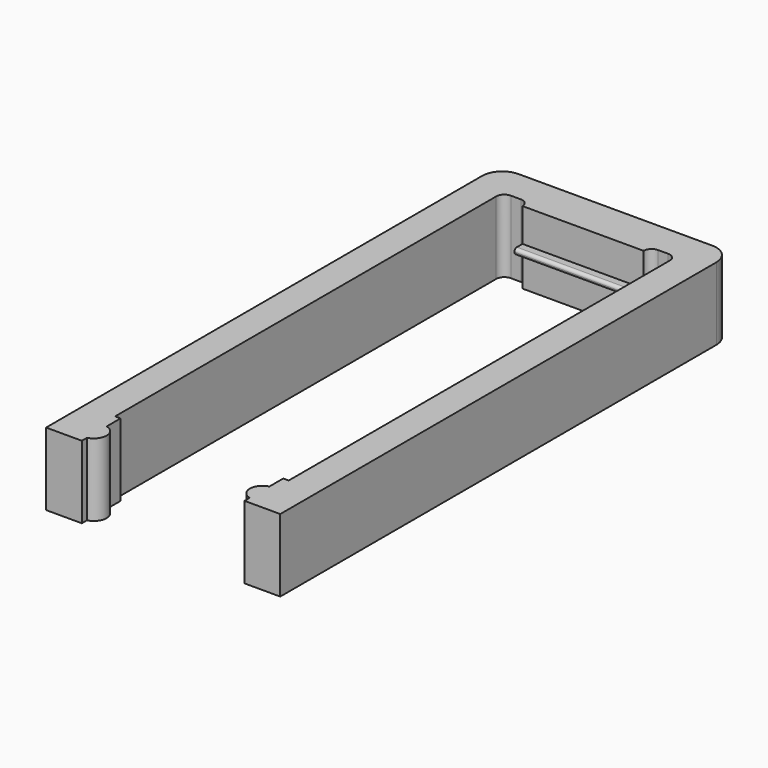
from build123d import *

# Parameters (mm, degrees)
F2_DEPTH = 18
F3_W     = 30
F3_H     = 1.5
F4_DEPTH = 2.5
F5_R     = 0.75
F6_R     = 0.74999


# Not quite as in the source:
# - a fillet or chamfer is up to 0.001 mm smaller than in the source, because OpenCascade refuses the exact size


with BuildPart() as f2:
    # F1 (on Top) → F2 (new body)
    with BuildSketch(Plane.XY):
        with BuildLine():
            Line((24, 140), (0, 140))
            Line((0, 140), (-24, 140))
            ThreePointArc((-24, 140), (-27.5355339059, 138.5355339059), (-29, 135))
            Line((-29, 135), (-29, 0))
            Line((-29, 0), (-20.15, 0))
            Line((-20.15, 0), (-20.15, 1.6))
            ThreePointArc((-20.15, 1.6), (-17.75, 4.65), (-20.15, 7.7))
            Line((-20.15, 7.7), (-20.15, 12))
            Line((-20.15, 12), (-21.5, 12))
            Line((-21.5, 12), (-21.5, 130))
            ThreePointArc((-21.5, 130), (-20.9142135624, 131.4142135624), (-19.5, 132))
            Line((-19.5, 132), (-17, 132))
            ThreePointArc((-17, 132), (-15.5857864376, 131.4142135624), (-15, 130))
            Line((-15, 130), (0, 130))
            Line((0, 130), (15, 130))
            ThreePointArc((15, 130), (15.5857864376, 131.4142135624), (17, 132))
            Line((17, 132), (19.5, 132))
            ThreePointArc((19.5, 132), (20.9142135624, 131.4142135624), (21.5, 130))
            Line((21.5, 130), (21.5, 12))
            Line((21.5, 12), (20.15, 12))
            Line((20.15, 12), (20.15, 7.7))
            ThreePointArc((20.15, 7.7), (17.75, 4.65), (20.15, 1.6))
            Line((20.15, 1.6), (20.15, 0))
            Line((20.15, 0), (29, 0))
            Line((29, 0), (29, 135))
            ThreePointArc((29, 135), (27.5355339059, 138.5355339059), (24, 140))
        make_face()
    extrude(amount=F2_DEPTH)

    # F3 (on face) → F4 (join)
    with BuildSketch(Plane.XZ.offset(-130)):
        with Locations((0, 9)):
            Rectangle(F3_W, F3_H)
    extrude(amount=F4_DEPTH)

    # F5
    f5_edges = [f2.edges().sort_by_distance(p)[0] for p in [
        (0, 127.5, 9.75),
    ]]
    fillet(f5_edges, radius=F5_R)

    # F6 (radius 0.75 in the source; OpenCascade refuses exactly that, so slightly less here)
    f6_edges = [f2.edges().sort_by_distance(p)[0] for p in [
        (0, 127.5, 8.25),
    ]]
    fillet(f6_edges, radius=F6_R)


solid = f2.part
